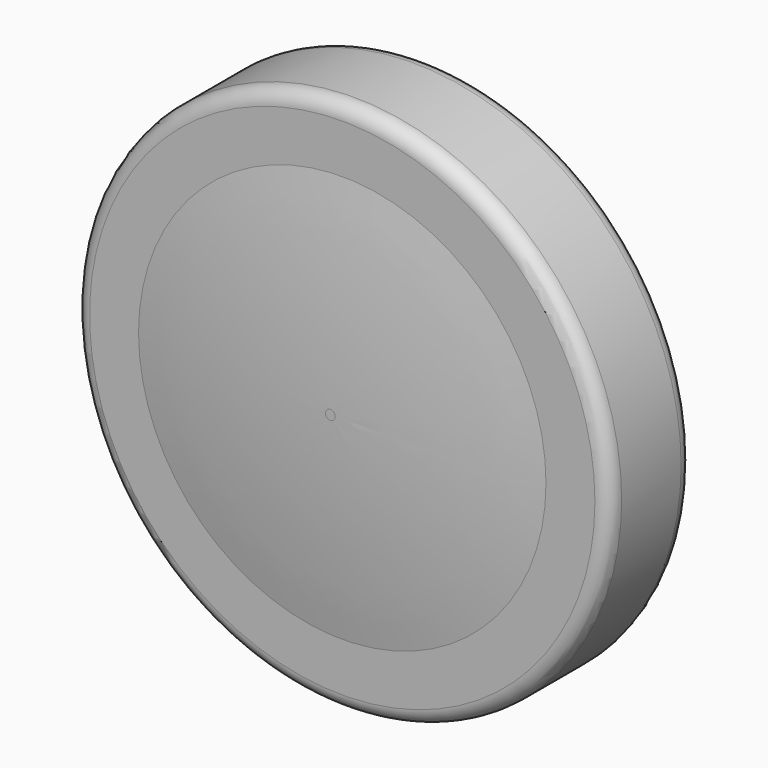
from build123d import *

# Parameters (mm, degrees)
F0_R     = 18
F0_R_2   = 13.6738896343
F1_DEPTH = 7
F2_R     = 1
F3_R     = 13.7073607276
F4_DEPTH = 8


# Not quite as in the source:
# - a fillet or chamfer that OpenCascade refuses, or shapes differently, is made with other operations: its cross-section is extruded or revolved along the edge and cut away or added


with BuildPart() as f1:
    # F0 (on Front) → F1 (new body)
    with BuildSketch(Plane.XZ):
        Circle(F0_R)
        Circle(F0_R_2, mode=Mode.SUBTRACT)
    extrude(amount=F1_DEPTH)

    # F2
    f2_edges = [f1.edges().sort_by_distance(p)[0] for p in [
        (-18, -7, 0),
        (-18, 0, 0),
    ]]
    fillet(f2_edges, radius=F2_R)

    # F3 (on Front) → F4 (join)
    with BuildSketch(Plane.XZ):
        Circle(F3_R)
    extrude(amount=F4_DEPTH)

    # F5: fillet of radius 90 on 1 edges, made by hand

    # F5_s1 → F5_t2 (revolve, cut)
    with BuildSketch(Plane.XY):
        with BuildLine():
            ThreePointArc((13.7073607276, -7), (7.0364764999, -7.7496518099), (0.3282725674, -8))
            Line((0.3282725674, -8), (13.7073607276, -8))
            Line((13.7073607276, -8), (13.7073607276, -7))
        make_face()
    revolve(axis=Axis((0, -8, 0), (0, -1, 0)), mode=Mode.SUBTRACT)


solid = f1.part
